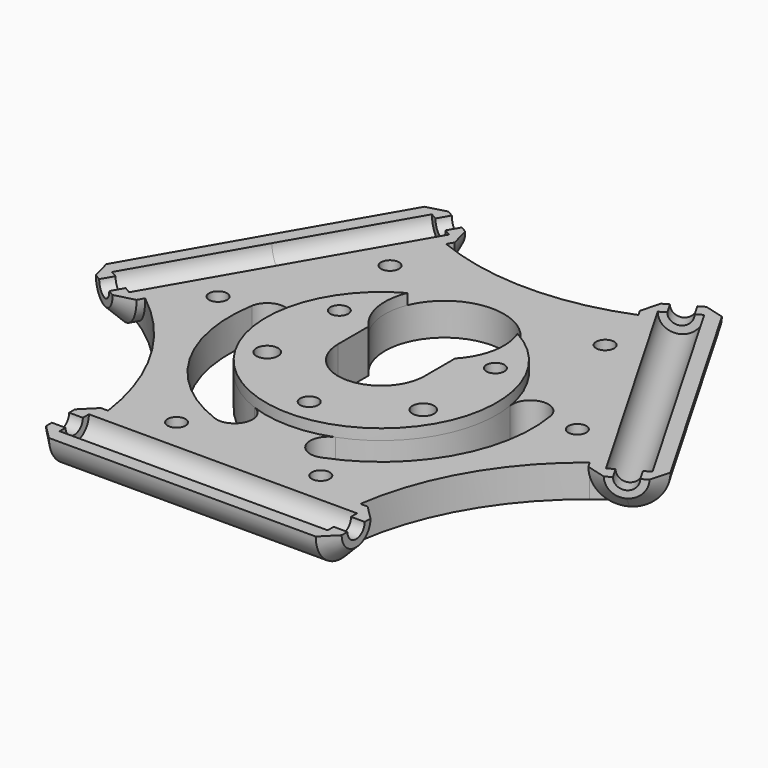
from build123d import *

# Parameters (mm, degrees)
F0_R            = 1.25
F0_R_2          = 1.5
F1_DEPTH        = 4.5
F2_R            = 1.5
F3_DEPTH        = 70.8788764306
F3_COPIES_COUNT = 3
F5_R            = 2.55
F6_DEPTH        = 18.6
F6_DEPTH_BACK   = 18.6
F6_COPIES_COUNT = 3
F8_T1_DEPTH     = 63.5
F8_T3_DEPTH     = 63.5
F8_T5_DEPTH     = 63.5
F8_T10_DEPTH    = 25.5
F8_S11_R        = 35.5
F8_T12_DEPTH    = 16
F8_T16_DEPTH    = 25.5
F8_S17_R        = 35.5
F8_T18_DEPTH    = 16
F8_T22_DEPTH    = 25.5
F8_S23_R        = 35.5
F8_T24_DEPTH    = 15
F8_T28_DEPTH    = 25.5
F8_S29_R        = 35.5
F8_T30_DEPTH    = 15
F8_T34_DEPTH    = 25.5
F8_S35_R        = 35.5
F8_T36_DEPTH    = 16
F8_T40_DEPTH    = 25.5
F8_S41_R        = 35.5
F8_T42_DEPTH    = 16
F9_SIZE         = 2
F10_R           = 1.5
F10_R_2         = 1.25
F11_DEPTH       = 1.5


# Not quite as in the source:
# - a fillet or chamfer that OpenCascade refuses, or shapes differently, is made with other operations: its cross-section is extruded or revolved along the edge and cut away or added
# - a pattern or mirror of a feature is missing from the dataset's text; its kind, count and spacing are read off the source's solid


with BuildPart() as f1:
    # F0 (on Top) → F1 (new body)
    with BuildSketch(Plane.XY):
        with BuildLine():
            Line((-40.1278764306, -0.5035207776), (-32.3336477965, -5.0035207776))
            Line((-32.3336477965, -5.0035207776), (-30.8336477965, -2.4054445662))
            ThreePointArc((-30.8336477965, -2.4054445662), (-21.9158664068, -12.6531313695), (-17.5, -25.5))
            Line((-17.5, -25.5), (-20.5, -25.5))
            Line((-20.5, -25.5), (-20.5, -34.5))
            Line((-20.5, -34.5), (20.5, -34.5))
            Line((20.5, -34.5), (20.5, -25.5))
            Line((20.5, -25.5), (17.5, -25.5))
            ThreePointArc((17.5, -25.5), (21.9158664068, -12.6531313695), (30.8336477965, -2.4054445662))
            Line((30.8336477965, -2.4054445662), (32.3336477965, -5.0035207776))
            Line((32.3336477965, -5.0035207776), (40.1278764306, -0.5035207776))
            Line((40.1278764306, -0.5035207776), (19.6278764306, 35.0035207776))
            Line((19.6278764306, 35.0035207776), (11.8336477965, 30.5035207776))
            Line((11.8336477965, 30.5035207776), (13.3336477965, 27.9054445662))
            ThreePointArc((13.3336477965, 27.9054445662), (0, 25.306262739), (-13.3336477965, 27.9054445662))
            Line((-13.3336477965, 27.9054445662), (-11.8336477965, 30.5035207776))
            Line((-11.8336477965, 30.5035207776), (-19.6278764306, 35.0035207776))
            Line((-19.6278764306, 35.0035207776), (-40.1278764306, -0.5035207776))
        make_face()
        with Locations((-10, -23)):
            Circle(F0_R, mode=Mode.SUBTRACT)
        with BuildLine():
            ThreePointArc((-20.7162162162, 3.4406955231), (-17.8403933901, 5.4973051295), (-15.7837837838, 2.6214823033))
            ThreePointArc((-15.7837837838, 2.6214823033), (-13.8564064606, -8), (-5.6216216216, -14.9798988763))
            ThreePointArc((-5.6216216216, -14.9798988763), (-4.1593908006, -18.1988864541), (-7.3783783784, -19.6611172751))
            ThreePointArc((-7.3783783784, -19.6611172751), (-18.1865334795, -10.5), (-20.7162162162, 3.4406955231))
        make_face(mode=Mode.SUBTRACT)
        with Locations((-10.8253175473, -6.25)):
            Circle(F0_R_2, mode=Mode.SUBTRACT)
        with Locations((10, -23)):
            Circle(F0_R, mode=Mode.SUBTRACT)
        with Locations((0, -12.5)):
            Circle(F0_R, mode=Mode.SUBTRACT)
        with BuildLine():
            ThreePointArc((5.6216216216, -14.9798988763), (13.8564064606, -8), (15.7837837838, 2.6214823033))
            ThreePointArc((15.7837837838, 2.6214823033), (17.8403933901, 5.4973051295), (20.7162162162, 3.4406955231))
            ThreePointArc((20.7162162162, 3.4406955231), (18.1865334795, -10.5), (7.3783783784, -19.6611172751))
            ThreePointArc((7.3783783784, -19.6611172751), (4.1593908006, -18.1988864541), (5.6216216216, -14.9798988763))
        make_face(mode=Mode.SUBTRACT)
        with Locations((10.8253175473, -6.25)):
            Circle(F0_R_2, mode=Mode.SUBTRACT)
        with Locations((-24.918584287, 2.8397459622)):
            Circle(F0_R, mode=Mode.SUBTRACT)
        with Locations((-10.8253175473, 6.25)):
            Circle(F0_R, mode=Mode.SUBTRACT)
        with Locations((-14.918584287, 20.1602540378)):
            Circle(F0_R, mode=Mode.SUBTRACT)
        with BuildLine():
            ThreePointArc((6, 0), (0, -6), (-6, 0))
            Line((-6, 0), (-6, 5.2915026221))
            ThreePointArc((-6, 5.2915026221), (0, 19.2038784486), (6, 5.2915026221))
            Line((6, 5.2915026221), (6, 0))
        make_face(mode=Mode.SUBTRACT)
        with Locations((10.8253175473, 6.25)):
            Circle(F0_R, mode=Mode.SUBTRACT)
        with Locations((24.918584287, 2.8397459622)):
            Circle(F0_R, mode=Mode.SUBTRACT)
        with Locations((14.918584287, 20.1602540378)):
            Circle(F0_R, mode=Mode.SUBTRACT)
    extrude(amount=F1_DEPTH)

    # F2 (on face) → F3 (cut, through all)
    with BuildSketch(Plane(origin=(-10.25, -17.7535207776, 0), x_dir=(0.8660254038, -0.5, 0), z_dir=(-0.5, -0.8660254038, 0))):
        with Locations((-30, 4.5)):
            Circle(F2_R)
    f3 = extrude(amount=-F3_DEPTH, mode=Mode.SUBTRACT)

    # F3_copies: F3 ×3 about axis
    f3_copies_axis = Axis((0, 0, 0), (0, 0, 1))
    for i in range(1, F3_COPIES_COUNT):
        add(f3.rotate(f3_copies_axis, i * 360 / F3_COPIES_COUNT), mode=Mode.SUBTRACT)

    # F5 (on plane+point) → F6 (cut, two sides)
    with BuildSketch(Plane(origin=(0, 0, 0), x_dir=(0.8660254038, -0.5, 0), z_dir=(-0.5, -0.8660254038, 0))) as f6_sk:
        with Locations((-30, 4.5)):
            Circle(F5_R)
    f6 = extrude(amount=-F6_DEPTH, mode=Mode.SUBTRACT) + extrude(f6_sk.sketch, amount=F6_DEPTH_BACK, mode=Mode.SUBTRACT)

    # F6_copies: F6 ×3 about axis
    f6_copies_axis = Axis((0, 0, 0), (0, 0, 1))
    for i in range(1, F6_COPIES_COUNT):
        add(f6.rotate(f6_copies_axis, i * 360 / F6_COPIES_COUNT), mode=Mode.SUBTRACT)

    # F8: fillet of radius 4.5 on 9 edges, made by hand

    # F8_s2 → F8_t1 (cut)
    with BuildSketch(Plane(origin=(15.875, 27.4963065702, 0), x_dir=(0, 0, 1), z_dir=(-0.5, -0.8660254038, 0))):
        with BuildLine():
            ThreePointArc((4.5, 34.5), (1.3180194847, 33.1819805153), (0, 30))
            Line((0, 30), (0, 34.5))
            Line((0, 34.5), (4.5, 34.5))
        make_face()
    extrude(amount=F8_T1_DEPTH, mode=Mode.SUBTRACT)

    # F8_s4 → F8_t3 (cut)
    with BuildSketch(Plane.YZ.offset(-31.75)):
        with BuildLine():
            ThreePointArc((-30, 0), (-33.1819805153, 1.3180194847), (-34.5, 4.5))
            Line((-34.5, 4.5), (-34.5, 0))
            Line((-34.5, 0), (-30, 0))
        make_face()
    extrude(amount=F8_T3_DEPTH, mode=Mode.SUBTRACT)

    # F8_s6 → F8_t5 (cut)
    with BuildSketch(Plane(origin=(15.875, -27.4963065702, 0), x_dir=(0, 0, 1), z_dir=(-0.5, 0.8660254038, 0))):
        with BuildLine():
            ThreePointArc((0, 30), (1.3180194847, 33.1819805153), (4.5, 34.5))
            Line((4.5, 34.5), (0, 34.5))
            Line((0, 34.5), (0, 30))
        make_face()
    extrude(amount=F8_T5_DEPTH, mode=Mode.SUBTRACT)


with BuildPart() as f8_tool8:
    # F8_s9 → F8_t10 (new body)
    with BuildSketch(Plane(origin=(-15.875, -27.4963065702, 0), x_dir=(0, 0, 1), z_dir=(0.5, 0.8660254038, 0))):
        with BuildLine():
            ThreePointArc((0, -30), (1.3180194847, -26.8180194847), (4.5, -25.5))
            Line((4.5, -25.5), (0, -25.5))
            Line((0, -25.5), (0, -30))
        make_face()
    extrude(amount=F8_T10_DEPTH)

    # F8_s11 → F8_t12 (intersect, symmetric)
    with BuildSketch(Plane.XY.offset(2.2)):
        with Locations((-52.6597682412, -30.4031313695)):
            Circle(F8_S11_R)
    extrude(amount=F8_T12_DEPTH, both=True, mode=Mode.INTERSECT)


with BuildPart() as f1_1:
    add(f1.part)

    # F8_t7: cut F8_tool8
    add(f8_tool8.part, mode=Mode.SUBTRACT)


with BuildPart() as f8_tool14:
    # F8_s15 → F8_t16 (new body)
    with BuildSketch(Plane(origin=(3.125, 5.4126587737, 0), x_dir=(0, 0, 1), z_dir=(0.5, 0.8660254038, 0))):
        with BuildLine():
            ThreePointArc((0, -30), (1.3180194847, -26.8180194847), (4.5, -25.5))
            Line((4.5, -25.5), (0, -25.5))
            Line((0, -25.5), (0, -30))
        make_face()
    extrude(amount=F8_T16_DEPTH)

    # F8_s17 → F8_t18 (intersect, symmetric)
    with BuildSketch(Plane.XY.offset(2.2)):
        with Locations((0, 60.806262739)):
            Circle(F8_S17_R)
    extrude(amount=F8_T18_DEPTH, both=True, mode=Mode.INTERSECT)


with BuildPart() as f1_2:
    add(f1_1.part)

    # F8_t13: cut F8_tool14
    add(f8_tool14.part, mode=Mode.SUBTRACT)


with BuildPart() as f8_tool20:
    # F8_s21 → F8_t22 (new body)
    with BuildSketch(Plane.YZ.offset(-6.25)):
        with BuildLine():
            ThreePointArc((-30, 0), (-26.8180194847, 1.3180194847), (-25.5, 4.5))
            Line((-25.5, 4.5), (-25.5, 0))
            Line((-25.5, 0), (-30, 0))
        make_face()
    extrude(amount=-F8_T22_DEPTH)

    # F8_s23 → F8_t24 (intersect, symmetric)
    with BuildSketch(Plane.XY.offset(2.2)):
        with Locations((-52.6597682412, -30.4031313695)):
            Circle(F8_S23_R)
    extrude(amount=F8_T24_DEPTH, both=True, mode=Mode.INTERSECT)


with BuildPart() as f1_3:
    add(f1_2.part)

    # F8_t19: cut F8_tool20
    add(f8_tool20.part, mode=Mode.SUBTRACT)


with BuildPart() as f8_tool26:
    # F8_s27 → F8_t28 (new body)
    with BuildSketch(Plane.YZ.offset(31.75)):
        with BuildLine():
            ThreePointArc((-30, 0), (-26.8180194847, 1.3180194847), (-25.5, 4.5))
            Line((-25.5, 4.5), (-25.5, 0))
            Line((-25.5, 0), (-30, 0))
        make_face()
    extrude(amount=-F8_T28_DEPTH)

    # F8_s29 → F8_t30 (intersect, symmetric)
    with BuildSketch(Plane.XY.offset(2.2)):
        with Locations((52.6597682412, -30.4031313695)):
            Circle(F8_S29_R)
    extrude(amount=F8_T30_DEPTH, both=True, mode=Mode.INTERSECT)


with BuildPart() as f1_4:
    add(f1_3.part)

    # F8_t25: cut F8_tool26
    add(f8_tool26.part, mode=Mode.SUBTRACT)


with BuildPart() as f8_tool32:
    # F8_s33 → F8_t34 (new body)
    with BuildSketch(Plane(origin=(3.125, -5.4126587737, 0), x_dir=(0, 0, 1), z_dir=(0.5, -0.8660254038, 0))):
        with BuildLine():
            ThreePointArc((0, -30), (1.3180194847, -26.8180194847), (4.5, -25.5))
            Line((4.5, -25.5), (0, -25.5))
            Line((0, -25.5), (0, -30))
        make_face()
    extrude(amount=F8_T34_DEPTH)

    # F8_s35 → F8_t36 (intersect, symmetric)
    with BuildSketch(Plane.XY.offset(2.3)):
        with Locations((52.6597682412, -30.4031313695)):
            Circle(F8_S35_R)
    extrude(amount=F8_T36_DEPTH, both=True, mode=Mode.INTERSECT)


with BuildPart() as f1_5:
    add(f1_4.part)

    # F8_t31: cut F8_tool32
    add(f8_tool32.part, mode=Mode.SUBTRACT)


with BuildPart() as f8_tool38:
    # F8_s39 → F8_t40 (new body)
    with BuildSketch(Plane(origin=(-15.875, 27.4963065702, 0), x_dir=(0, 0, 1), z_dir=(0.5, -0.8660254038, 0))):
        with BuildLine():
            ThreePointArc((0, -30), (1.3180194847, -26.8180194847), (4.5, -25.5))
            Line((4.5, -25.5), (0, -25.5))
            Line((0, -25.5), (0, -30))
        make_face()
    extrude(amount=F8_T40_DEPTH)

    # F8_s41 → F8_t42 (intersect, symmetric)
    with BuildSketch(Plane.XY.offset(2.2)):
        with Locations((0, 60.806262739)):
            Circle(F8_S41_R)
    extrude(amount=F8_T42_DEPTH, both=True, mode=Mode.INTERSECT)


with BuildPart() as f1_6:
    add(f1_5.part)

    # F8_t37: cut F8_tool38
    add(f8_tool38.part, mode=Mode.SUBTRACT)

    # F9
    f9_edges = [f1_6.edges().sort_by_distance(p)[0] for p in [
        (-38.986438, -1.162531, 1.318019),
        (-20.5, -26.818019, 1.318019),
        (20.5, -33.181981, 1.318019),
        (33.475086, -4.344511, 1.318019),
        (-33.475086, -4.344511, 1.318019),
        (-18.486438, 34.344511, 1.318019),
        (-12.975086, 31.162531, 1.318019),
        (38.986438, -1.162531, 1.318019),
        (20.5, -26.818019, 1.318019),
        (-20.5, -33.181981, 1.318019),
        (12.975086, 31.162531, 1.318019),
        (18.486438, 34.344511, 1.318019),
    ]]
    chamfer(f9_edges, length=F9_SIZE)

    # F10 (on face) → F11 (join)
    with BuildSketch(Plane.XY.offset(4.5)):
        with BuildLine():
            ThreePointArc((-6, 5.2915026221), (-8.1084434906, 9.432154374), (-7.6447569596, 14.0555217274))
            ThreePointArc((-7.6447569596, 14.0555217274), (0, -16), (7.6447569596, 14.0555217274))
            ThreePointArc((7.6447569596, 14.0555217274), (8.1084434906, 9.432154374), (6, 5.2915026221))
            Line((6, 5.2915026221), (6, 0))
            ThreePointArc((6, 0), (0, -6), (-6, 0))
            Line((-6, 0), (-6, 5.2915026221))
        make_face()
        with Locations((-10.8253175473, -6.25)):
            Circle(F10_R, mode=Mode.SUBTRACT)
        with Locations((0, -12.5)):
            Circle(F10_R_2, mode=Mode.SUBTRACT)
        with Locations((10.8253175473, -6.25)):
            Circle(F10_R, mode=Mode.SUBTRACT)
        with Locations((-10.8253175473, 6.25)):
            Circle(F10_R_2, mode=Mode.SUBTRACT)
        with Locations((10.8253175473, 6.25)):
            Circle(F10_R_2, mode=Mode.SUBTRACT)
    extrude(amount=F11_DEPTH)


solid = f1_6.part
